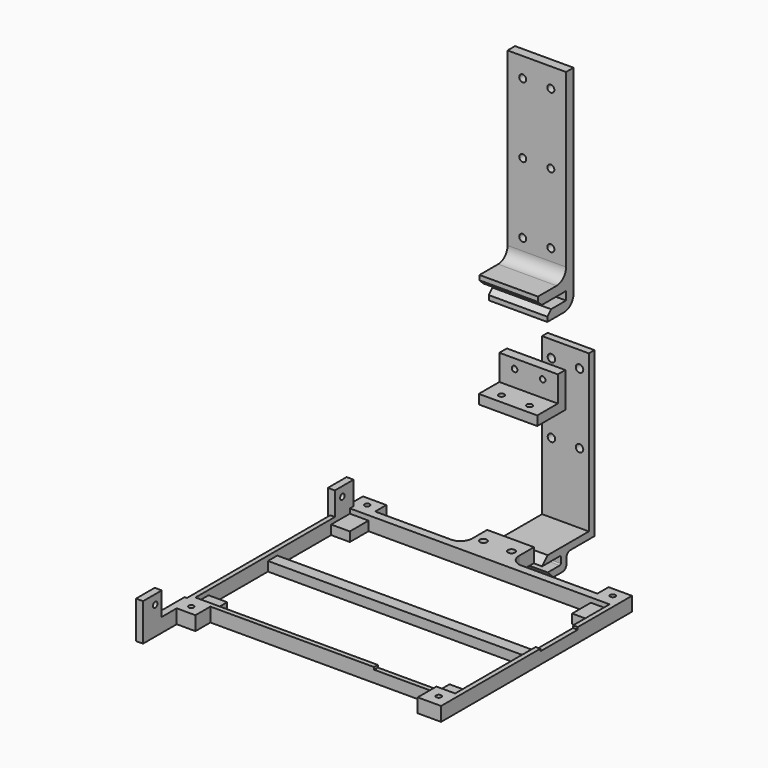
from build123d import *

# Parameters (mm, degrees)
F0_W             = 115
F0_H             = 86.5
F0_W_2           = 111
F0_H_2           = 82.5
F1_DEPTH         = 6
F2_W             = 8
F2_H             = 10
F2_H_2           = 7
F2_W_2           = 111
F2_H_3           = 5
F3_DEPTH         = 4
F4_W             = 25
F4_H             = 2
F4_W_2           = 2
F4_H_2           = 20
F5_DEPTH         = 1
F6_W             = 20
F6_H             = 13
F7_DEPTH         = 6
F8_W             = 20
F8_H             = 12
F9_DEPTH         = 3
F10_W            = 3
F10_H            = 70
F11_DEPTH        = 20
F12_W            = 3
F12_H            = 10
F12_H_2          = 26
F13_DEPTH        = 16
F14_SIZE         = 2.99999
F15_W            = 16
F15_H            = 10
F15_R            = 1.2
F16_DEPTH        = 25
F17_R            = 2
F18_W            = 4
F18_H            = 11
F19_DEPTH        = 12.5
F22_D            = 2.4
F22_DEPTH        = 5
F22_TIP          = 0.7210327428
F22_ON_F21_D     = 2.4
F22_ON_F21_DEPTH = 5
F22_ON_F21_TIP   = 0.7210327428
F23_R            = 1.6
F24_DEPTH        = 25
F26_DEPTH        = 12.5
F27_R            = 5
F27_2_R          = 5
F28_SIZE         = 2
F29_R            = 1.5
F30_DEPTH        = 25
F31_W            = 10
F31_H            = 6
F31_H_2          = 8
F31_W_2          = 8
F32_DEPTH        = 6
F33_R            = 1.1
F33_R_2          = 1.5
F34_DEPTH        = 2


# Not quite as in the source:
# - a fillet or chamfer is up to 0.001 mm smaller than in the source, because OpenCascade refuses the exact size


with BuildPart() as f1:
    # F0 (on Top) → F1 (new body)
    with BuildSketch(Plane.XY):
        Rectangle(F0_W, F0_H)
        Rectangle(F0_W_2, F0_H_2, mode=Mode.SUBTRACT)
    extrude(amount=F1_DEPTH)

    # F2 (on face) → F3 (join)
    with BuildSketch(Plane(origin=(0, 0, 0), x_dir=(1, 0, 0), z_dir=(0, 0, -1))):
        with Locations((-51.5, -36.25)):
            Rectangle(F2_W, F2_H)
        with Locations((51.5, -36.25)):
            Rectangle(F2_W, F2_H)
        with Locations((-51.5, 37.75)):
            Rectangle(F2_W, F2_H_2)
        with Locations((51.5, 37.75)):
            Rectangle(F2_W, F2_H_2)
        Rectangle(F2_W_2, F2_H_3)
    extrude(amount=-F3_DEPTH)

    # F4 (on face) → F5 (cut)
    with BuildSketch(Plane.XY.offset(6)):
        with Locations((35, -42.25)):
            Rectangle(F4_W, F4_H)
        with Locations((56.5, 11.75)):
            Rectangle(F4_W_2, F4_H_2)
    extrude(amount=-F5_DEPTH, mode=Mode.SUBTRACT)

    # F6 (on face) → F7 (join)
    with BuildSketch(Plane(origin=(0, 0, 0), x_dir=(1, 0, 0), z_dir=(0, 0, -1))):
        with Locations((0, -51.25)):
            Rectangle(F6_W, F6_H)
        Polygon((-10, -44.75), (10, -44.75), (57.5, -44.75), (57.5, -43.25), (-57.5, -43.25), (-57.5, -44.75), align=None)
    extrude(amount=-F7_DEPTH)

    # F12 (on Top) → F13 (join)
    with BuildSketch(Plane.XY):
        with Locations((-57, 38.25)):
            Rectangle(F12_W, F12_H)
        with Locations((-57, -56.25)):
            Rectangle(F12_W, F12_H_2)
    extrude(amount=F13_DEPTH)

    # F15 (on face) → F16 (cut)
    with BuildSketch(Plane.YZ.offset(-55.5)):
        with Locations((-51.25, 11)):
            Rectangle(F15_W, F15_H)
        with Locations((-62.75, 12)):
            Circle(F15_R)
        with Locations((37.25, 12)):
            Circle(F15_R)
    extrude(amount=-F16_DEPTH, mode=Mode.SUBTRACT)

    # F27
    f27_edges = [f1.edges().sort_by_distance(p)[0] for p in [
        (-10, 44.75, 3),
        (10, 44.75, 3),
    ]]
    fillet(f27_edges, radius=F27_R)

    # F31 (on Top) → F32 (join)
    with BuildSketch(Plane.XY):
        with Locations((-52.5, 47.75)):
            Rectangle(F31_W, F31_H)
        with Locations((52.5, 47.75)):
            Rectangle(F31_W, F31_H)
        with Locations((52.5, -47.25)):
            Rectangle(F31_W, F31_H_2)
        with Locations((-51.5, -47.25)):
            Rectangle(F31_W_2, F31_H_2)
    extrude(amount=F32_DEPTH)

    # F33 (on face) → F34 (cut)
    with BuildSketch(Plane.XY.offset(6)):
        with Locations((-52.5, 46.75)):
            Circle(F33_R)
        with Locations((52.5, 46.75)):
            Circle(F33_R)
        with Locations((-52.5, -47.25)):
            Circle(F33_R)
        with Locations((52.5, -46.25)):
            Circle(F33_R)
        with Locations((-6, 50.75)):
            Circle(F33_R_2)
        with Locations((6, 50.75)):
            Circle(F33_R_2)
    extrude(amount=-F34_DEPTH, mode=Mode.SUBTRACT)


with BuildPart() as f9:
    # F8 (on Top) → F9 (new body)
    with BuildSketch(Plane.XY):
        with Locations((0, 81.0819491744)):
            Rectangle(F8_W, F8_H)
    extrude(amount=-F9_DEPTH)

    # F10 (on face) → F11 (join)
    with BuildSketch(Plane(origin=(-10, 0, 0), x_dir=(0, -1, 0), z_dir=(-1, 0, 0))):
        with BuildLine():
            Line((-75.0819491744, 0), (-75.0819491744, -3))
            Line((-75.0819491744, -3), (-75.0819491744, -9.5))
            Line((-75.0819491744, -9.5), (-65.0819491744, -9.5))
            Line((-65.0819491744, -9.5), (-65.0819491744, -6.5))
            Line((-65.0819491744, -6.5), (-71.5819491744, -6.5))
            ThreePointArc((-71.5819491744, -6.5), (-71.935502565, -6.3535533906), (-72.0819491744, -6))
            Line((-72.0819491744, -6), (-72.0819491744, -3.5))
            ThreePointArc((-72.0819491744, -3.5), (-71.935502565, -3.1464466094), (-71.5819491744, -3))
            Line((-71.5819491744, -3), (-62.0819491744, -3))
            Line((-62.0819491744, -3), (-62.0819491744, 0))
            Line((-62.0819491744, 0), (-75.0819491744, 0))
        make_face()
        with Locations((-88.5819491744, 32)):
            Rectangle(F10_W, F10_H)
    extrude(amount=-F11_DEPTH)

    # F14 (size 3 in the source; OpenCascade refuses exactly that, so slightly less here)
    f14_edges = [f9.edges().sort_by_distance(p)[0] for p in [
        (0, 62.081949, 0),
        (0, 65.081949, -9.5),
    ]]
    chamfer(f14_edges, length=F14_SIZE)

    # F17
    f17_edges = [f9.edges().sort_by_distance(p)[0] for p in [
        (0, 75.081949, -3),
        (0, 75.081949, -9.5),
    ]]
    fillet(f17_edges, radius=F17_R)

    # F23 (on face) → F24 (cut)
    with BuildSketch(Plane(origin=(0, 90.0819491744, 0), x_dir=(-1, 0, 0), z_dir=(0, 1, 0))):
        with Locations((-6, 30)):
            Circle(F23_R)
        with Locations((6, 30)):
            Circle(F23_R)
        with Locations((-6, 60)):
            Circle(F23_R)
        with Locations((6, 60)):
            Circle(F23_R)
    extrude(amount=-F24_DEPTH, mode=Mode.SUBTRACT)


with BuildPart() as f19:
    # F18 (on Right) → F19 (new body, symmetric)
    with BuildSketch(Plane.YZ):
        Polygon((67.3785170999, 56.9265080243), (56.3785170999, 56.9265080243), (56.3785170999, 52.9265080243), (71.3785170999, 52.9265080243), (71.3785170999, 56.9265080243), align=None)
        with Locations((69.3785170999, 62.4265080243)):
            Rectangle(F18_W, F18_H)
    extrude(amount=F19_DEPTH, both=True)

    # F22
    with Locations(Plane.XY.offset(56.9265080243)):
        with Locations((-6, 60.3785170999), (6, 60.3785170999)):
            Hole(F22_D / 2, depth=F22_DEPTH)
            with Locations((0, 0, -(F22_DEPTH + F22_TIP / 2))):  # 118° drill point
                Cone(0, F22_D / 2, F22_TIP, mode=Mode.SUBTRACT)

    # F22 on F21
    with Locations(Plane.XZ.offset(-67.3785170999)):
        with Locations((-6, 63.9265080243), (6, 63.9265080243)):
            Hole(F22_ON_F21_D / 2, depth=F22_ON_F21_DEPTH)
            with Locations((0, 0, -(F22_ON_F21_DEPTH + F22_ON_F21_TIP / 2))):  # 118° drill point
                Cone(0, F22_ON_F21_D / 2, F22_ON_F21_TIP, mode=Mode.SUBTRACT)


with BuildPart() as f26:
    # F25 (on Right) → F26 (new body, symmetric)
    with BuildSketch(Plane.YZ):
        Polygon((61.7522996068, 93.9075465441), (61.7522996068, 89.9075465441), (75.7522996068, 89.9075465441), (75.7522996068, 179.9075465441), (71.7522996068, 179.9075465441), (71.7522996068, 101.5075465441), (56.7522996068, 101.5075465441), (56.7522996068, 97.5075465441), (71.7522996068, 97.5075465441), (71.7522996068, 93.9075465441), align=None)
    extrude(amount=F26_DEPTH, both=True)

    # F27#2
    f27_2_edges = [f26.edges().sort_by_distance(p)[0] for p in [
        (0, 71.7523, 101.507547),
        (0, 75.7523, 89.907547),
    ]]
    fillet(f27_2_edges, radius=F27_2_R)

    # F28
    f28_edges = [f26.edges().sort_by_distance(p)[0] for p in [
        (0, 56.7523, 97.507547),
        (0, 61.7523, 93.907547),
    ]]
    chamfer(f28_edges, length=F28_SIZE)

    # F29 (on face) → F30 (cut)
    with BuildSketch(Plane(origin=(0, 75.7522996068, 0), x_dir=(-1, 0, 0), z_dir=(0, 1, 0))):
        with Locations((6, 111.5075465441)):
            Circle(F29_R)
        with Locations((-6, 111.5075465441)):
            Circle(F29_R)
        with Locations((6, 141.5075465441)):
            Circle(F29_R)
        with Locations((-6, 141.5075465441)):
            Circle(F29_R)
        with Locations((6, 171.5075465441)):
            Circle(F29_R)
        with Locations((-6, 171.5075465441)):
            Circle(F29_R)
    extrude(amount=-F30_DEPTH, mode=Mode.SUBTRACT)


solid = Compound([f1.part, f9.part, f19.part, f26.part])
